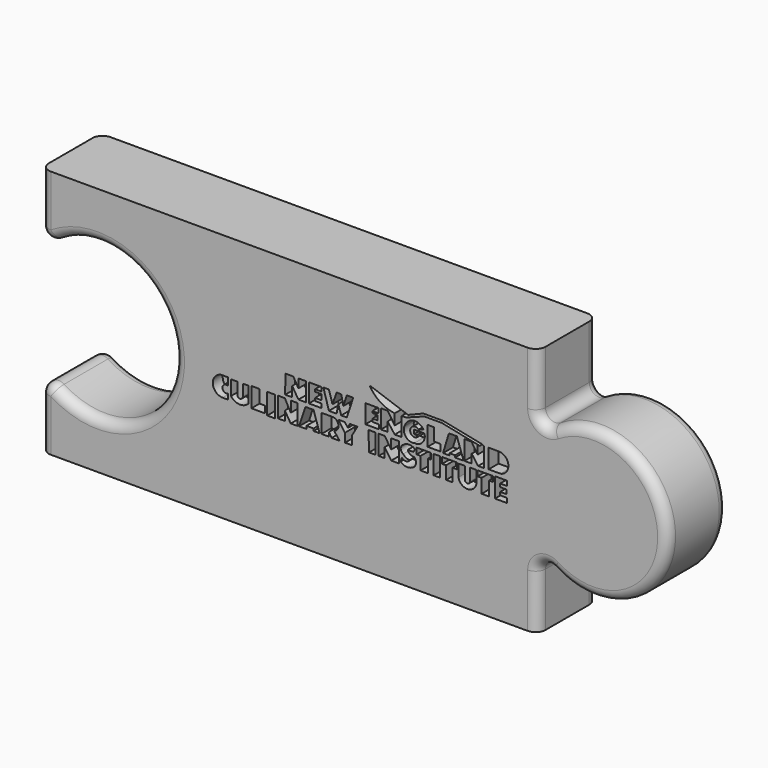
from build123d import *

# Parameters (mm, degrees)
F0_W     = 4.1021890939
F0_H     = 10.701617226
F0_W_2   = 3.2950267196
F0_H_2   = 9.6638526741
F1_DEPTH = 38.1
F2_W     = 160.8449816704
F2_H     = 39.124455303
F3_DEPTH = 31.75
F4_F1_R  = 5.08
F4_F2_R  = 5.08


with BuildPart() as f1:
    # F0 (on Front) → F1 (new body)
    with BuildSketch(Plane.XZ):
        with BuildLine():
            Line((82.5877203729, 87.3429829219), (-171.4122796271, 87.3429829219))
            Line((-171.4122796271, 87.3429829219), (-171.4122796271, 50.2589829219))
            ThreePointArc((-171.4122796271, 50.2589829219), (-103.0818238296, 23.5889829219), (-171.4122796271, -3.0810170781))
            Line((-171.4122796271, -3.0810170781), (-171.4122796271, -40.1650170781))
            Line((-171.4122796271, -40.1650170781), (82.5877203729, -40.1650170781))
            Line((82.5877203729, -40.1650170781), (82.5877203729, -1.8110170781))
            ThreePointArc((82.5877203729, -1.8110170781), (149.0857836871, 23.5889829219), (82.5877203729, 48.9889829219))
            Line((82.5877203729, 48.9889829219), (82.5877203729, 87.3429829219))
        make_face()
        with BuildLine():
            Line((-79.1224884233, 24.1685174963), (-75.8061008891, 24.1685174963))
            Line((-75.8061008891, 24.1685174963), (-75.8061008891, 20.3344915619))
            ThreePointArc((-75.8061008891, 20.3344915619), (-78.5705902931, 18.5480085759), (-75.8061008891, 16.7615255898))
            Line((-75.8061008891, 16.7615255898), (-75.8061008891, 14.1044995373))
            Line((-75.8061008891, 14.1044995373), (-78.4734087428, 14.1044995373))
            ThreePointArc((-78.4734087428, 14.1044995373), (-83.5158724737, 18.8322256207), (-79.1224884233, 24.1685174963))
        make_face(mode=Mode.SUBTRACT)
        with BuildLine():
            Line((-74.1997333607, 16.2316384351), (-74.1997333607, 23.7863697669))
            Line((-74.1997333607, 23.7863697669), (-70.9757404765, 23.7863697669))
            Line((-70.9757404765, 23.7863697669), (-70.9757404765, 18.0120524576))
            ThreePointArc((-70.9757404765, 18.0120524576), (-69.6300867408, 16.5195255788), (-68.1848200402, 17.9158151707))
            Line((-68.1848200402, 17.9158151707), (-68.1848200402, 23.7863697669))
            Line((-68.1848200402, 23.7863697669), (-65.2976604542, 23.7863697669))
            Line((-65.2976604542, 23.7863697669), (-65.2976604542, 15.654207263))
            ThreePointArc((-65.2976604542, 15.654207263), (-69.8819719959, 13.8882631575), (-74.1997333607, 16.2316384351))
        make_face(mode=Mode.SUBTRACT)
        Polygon((-63.7486102423, 14.098005425), (-63.7486102423, 24.1685174963), (-59.7253116211, 24.1685174963), (-59.7253116211, 17.5690884328), (-56.8064423642, 17.5690884328), (-56.8064423642, 14.098005425), align=None, mode=Mode.SUBTRACT)
        with Locations((-53.6509184531, 18.8177088833)):
            Rectangle(F0_W, F0_H, mode=Mode.SUBTRACT)
        Polygon((-46.6518933317, 13.9632076582), (-50.2579296371, 13.9632076582), (-50.2579296371, 24.2781453392), (-46.6518933317, 24.1685174963), (-43.6328882715, 18.6594389936), (-43.6328882715, 24.1685174963), (-40.2784357211, 24.1685174963), (-40.2784357211, 13.7954857758), (-43.6328882715, 13.7954857758), (-46.6518933317, 18.6594389936), align=None, mode=Mode.SUBTRACT)
        Polygon((-31.9960760316, 15.3444652072), (-35.6157990536, 15.3947389311), (-35.6157990536, 13.93679535), (-39.3863441786, 13.93679535), (-36.1185381553, 23.7402115574), (-31.9960760316, 23.7402115574), (-28.8790921113, 14.1881649008), (-31.9960760316, 14.1881649008), align=None, mode=Mode.SUBTRACT)
        with BuildLine():
            Line((-22.6569390288, 14.1316857746), (-24.1320217392, 16.3264675623))
            Line((-24.1320217392, 16.3264675623), (-24.1320217392, 14.2231351322))
            Line((-24.1320217392, 14.2231351322), (-27.91932322, 14.2231351322))
            Line((-27.91932322, 14.2231351322), (-27.91932322, 23.7338562122))
            Line((-27.91932322, 23.7338562122), (-22.2911415985, 23.7338562122))
            ThreePointArc((-22.2911415985, 23.7338562122), (-19.2453874648, 21.0752446961), (-21.4680983117, 17.6982060632))
            Line((-21.4680983117, 17.6982060632), (-18.633171021, 14.1316857746))
            Line((-18.633171021, 14.1316857746), (-22.6569390288, 14.1316857746))
        make_face(mode=Mode.SUBTRACT)
        Polygon((-15.9811424455, 14.1316857746), (-15.9811424455, 18.6126977763), (-19.3647658816, 23.4595090708), (-16.0725927344, 23.4595090708), (-14.3805118641, 21.3320423475), (-13.4205641589, 23.4595090708), (-9.48824644, 23.4595090708), (-12.3231737307, 18.7041480651), (-12.3231737307, 14.2231351322), align=None, mode=Mode.SUBTRACT)
        Polygon((-0.3251792295, 13.8158174789), (-3.5847491017, 13.8158174789), (-3.927862308, 23.8518603703), (-0.3251792295, 23.8518603703), align=None, mode=Mode.SUBTRACT)
        Polygon((4.3926183935, 13.8158174789), (1.3046059394, 13.8158174789), (1.1330493362, 23.8518603703), (4.3926183935, 23.8518603703), (7.7379672657, 18.7909491917), (7.7379672657, 23.8518603703), (11.6837615715, 23.8518603703), (11.6837615715, 13.8158174789), (7.7379672657, 13.8158174789), (4.3926183935, 18.7909491917), align=None, mode=Mode.SUBTRACT)
        with BuildLine():
            ThreePointArc((18.0667647728, 13.9566269329), (15.1280441908, 13.6247220185), (12.455818207, 14.8917846939))
            Line((12.455818207, 14.8917846939), (13.2156335385, 16.9374421796))
            ThreePointArc((13.2156335385, 16.9374421796), (15.2956200346, 15.9580622779), (17.2485019648, 17.1712320855))
            ThreePointArc((17.2485019648, 17.1712320855), (15.3278375039, 17.5219921442), (13.8585548484, 18.8077577016))
            ThreePointArc((13.8585548484, 18.8077577016), (12.5974932093, 20.8534151873), (13.8585548484, 22.899072673))
            ThreePointArc((13.8585548484, 22.899072673), (16.8685940662, 24.0004192145), (19.878633284, 22.899072673))
            Line((19.878633284, 22.899072673), (19.1772654289, 21.3794410786))
            Line((19.1772654289, 21.3794410786), (16.1380022401, 21.3794410786))
            ThreePointArc((16.1380022401, 21.3794410786), (17.4509312815, 19.7687555595), (19.4695023456, 19.2753375134))
            ThreePointArc((19.4695023456, 19.2753375134), (20.2970090792, 16.2127620999), (18.0667647728, 13.9566269329))
        make_face(mode=Mode.SUBTRACT)
        Polygon((22.741639019, 20.7961425743), (20.6964490572, 20.7961425743), (20.6964490572, 23.9033129597), (28.0818557003, 23.9033129597), (28.0818557003, 20.7961425743), (26.4911530176, 20.7961425743), (26.4911530176, 14.2394602856), (22.741639019, 14.2394602856), align=None, mode=Mode.SUBTRACT)
        with Locations((31.0928290346, 19.0713866227)):
            Rectangle(F0_W_2, F0_H_2, mode=Mode.SUBTRACT)
        Polygon((39.1031568506, 14.2394602856), (35.8081282684, 14.2394602856), (35.7312550405, 20.7961425743), (33.7629383066, 20.7961425743), (33.7629383066, 23.8972995988), (41.375587658, 23.8972995988), (41.375587658, 20.7961425743), (39.1031568506, 20.7961425743), align=None, mode=Mode.SUBTRACT)
        with BuildLine():
            Line((42.1253582099, 17.4266091174), (42.1253582099, 23.6942507884))
            Line((42.1253582099, 23.6942507884), (45.3586643198, 23.6942507884))
            Line((45.3586643198, 23.6942507884), (45.3586643198, 17.4266091174))
            ThreePointArc((45.3586643198, 17.4266091174), (46.7496648507, 16.1821081418), (48.0447960654, 17.5260948575))
            Line((48.0447960654, 17.5260948575), (48.0447960654, 23.7937365285))
            Line((48.0447960654, 23.7937365285), (51.2781021753, 23.7937365285))
            Line((51.2781021753, 23.7937365285), (51.2781021753, 17.5260948575))
            ThreePointArc((51.2781021753, 17.5260948575), (46.7430544325, 13.674498706), (42.1253582099, 17.4266091174))
        make_face(mode=Mode.SUBTRACT)
        Polygon((51.9394976655, 21.0886225662), (51.9394976655, 23.8059256783), (59.7690110663, 23.8059256783), (59.7690110663, 21.0886225662), (57.7886020401, 21.0886225662), (57.7886020401, 13.9038926548), (53.9659587303, 13.9038926548), (53.9659587303, 21.0886225662), align=None, mode=Mode.SUBTRACT)
        Polygon((60.7447465518, 13.9480652845), (60.7447465518, 24.0340419671), (63.44380878, 24.0340419671), (66.853153483, 24.0340419671), (66.853153483, 21.6190908661), (63.44380878, 21.6190908661), (63.44380878, 19.9854467621), (66.7111007133, 19.9854467621), (66.7111007133, 17.8546067885), (63.44380878, 17.8546067885), (63.44380878, 16.2919900006), (67.066240088, 16.2919900006), (67.066240088, 13.9480652845), (63.44380878, 13.9480652845), align=None, mode=Mode.SUBTRACT)
        Polygon((-42.9098839304, 25.8483980408), (-46.4937063298, 25.8483980408), (-46.4062684024, 35.39024299), (-42.3295787778, 35.39024299), (-39.7238294026, 30.8894083646), (-39.7238294026, 35.39024299), (-35.9475324294, 35.39024299), (-35.9475324294, 25.8483980408), (-39.7238294026, 25.8483980408), (-42.9098839304, 30.9736058673), align=None, mode=Mode.SUBTRACT)
        Polygon((-34.3518639347, 25.8483980408), (-34.3518639347, 35.39024299), (-27.91932322, 35.39024299), (-27.91932322, 33.288311269), (-31.2072942397, 33.288311269), (-31.2072942397, 32.140087392), (-27.91932322, 32.140087392), (-27.91932322, 29.3885917029), (-31.2072942397, 29.3885917029), (-31.2072942397, 27.9473327658), (-27.91932322, 27.9473327658), (-27.91932322, 25.8483980408), align=None, mode=Mode.SUBTRACT)
        Polygon((-20.2013133457, 25.8483980408), (-24.1320217392, 25.8483980408), (-26.9724550089, 35.4833715221), (-24.1320217392, 35.4833715221), (-22.2976906589, 29.3885917029), (-20.2013133457, 35.39024299), (-17.8428879371, 35.39024299), (-16.7425917825, 30.4357428661), (-14.959094151, 35.8198807201), (-11.6949612638, 35.8198807201), (-14.959094151, 25.8483980408), (-17.8428879371, 25.8483980408), (-19.3337081364, 30.4357428661), align=None, mode=Mode.SUBTRACT)
        Polygon((-5.4699555403, 25.8483980408), (-5.4699555403, 35.39024299), (1.1757765533, 35.39024299), (1.1757765533, 32.9699069819), (-1.9255653387, 32.9699069819), (-1.9255653387, 32.0838094315), (0.6219655843, 32.0838094315), (0.6219655843, 29.6470411679), (-1.8148031449, 29.6470411679), (-1.8148031449, 28.0963704547), (1.5080631347, 28.0963704547), (1.5080631347, 25.8483980408), align=None, mode=Mode.SUBTRACT)
        with BuildLine():
            Line((24.2475764846, 33.265524262), (21.7615682268, 32.337741982))
            ThreePointArc((21.7615682268, 32.337741982), (19.2187327571, 32.9434510536), (17.4847645322, 30.987370815))
            ThreePointArc((17.4847645322, 30.987370815), (18.327813662, 28.655644589), (20.8024000385, 28.5003986767))
            Line((20.8024000385, 28.5003986767), (20.8024000385, 29.5222215912))
            Line((20.8024000385, 29.5222215912), (19.4784858832, 29.5222215912))
            Line((19.4784858832, 29.5222215912), (19.4784858832, 31.5818060747))
            Line((19.4784858832, 31.5818060747), (24.7486075023, 31.5818060747))
            ThreePointArc((24.7486075023, 31.5818060747), (23.7703698462, 27.2257006882), (19.6384498486, 25.5345944872))
            ThreePointArc((19.6384498486, 25.5345944872), (15.2144546519, 26.9788151616), (14.5289026769, 31.5818060747))
            ThreePointArc((14.5289026769, 31.5818060747), (16.4834400671, 34.3767192692), (19.6384498486, 35.6719680688))
            ThreePointArc((19.6384498486, 35.6719680688), (22.2010175105, 34.9629088341), (24.2475764846, 33.265524262))
        make_face(mode=Mode.SUBTRACT)
        with BuildLine():
            ThreePointArc((9.5256541026, 35.6719680688), (2.0934573821, 38.3433933505), (-3.3327658093, 44.0818742475))
            Line((-3.3327658093, 44.0818742475), (16.3243263596, 37.1917598507))
            Line((16.3243263596, 37.1917598507), (24.1828551152, 40.3606482407))
            Line((24.1828551152, 40.3606482407), (34.1483158627, 40.3606482407))
            Line((34.1483158627, 40.3606482407), (54.2648797491, 36.2813287041))
            Line((54.2648797491, 36.2813287041), (55.0723811248, 35.6719680688))
            Line((55.0723811248, 35.6719680688), (55.0723811248, 25.8483980408))
            Line((55.0723811248, 25.8483980408), (52.1580790737, 25.8483980408))
            Line((52.1580790737, 25.8483980408), (48.8858809331, 30.2965418062))
            Line((48.8858809331, 30.2965418062), (48.8858809331, 25.8483980408))
            Line((48.8858809331, 25.8483980408), (45.2046608189, 25.8483980408))
            Line((45.2046608189, 25.8483980408), (45.2046608189, 35.6719680688))
            Line((45.2046608189, 35.6719680688), (48.820163087, 35.6719680688))
            Line((48.820163087, 35.6719680688), (51.9061637679, 30.8592357299))
            Line((51.9061637679, 30.8592357299), (51.9061637679, 35.171344932))
            Line((51.9061637679, 35.171344932), (53.0161512652, 35.171344932))
            Line((53.0161512652, 35.171344932), (33.7054067859, 39.1795598528))
            Line((33.7054067859, 39.1795598528), (24.6995845446, 39.1795598528))
            Line((24.6995845446, 39.1795598528), (15.3009332353, 35.6719680688))
            Line((15.3009332353, 35.6719680688), (13.1191615583, 35.6719680688))
            Line((13.1191615583, 35.6719680688), (13.1191615583, 26.110673379))
            Line((13.1191615583, 26.110673379), (9.5256541026, 26.110673379))
            Line((9.5256541026, 26.110673379), (5.9321474619, 30.8592357299))
            Line((5.9321474619, 30.8592357299), (5.9321474619, 26.110673379))
            Line((5.9321474619, 26.110673379), (2.4669798659, 26.110673379))
            Line((2.4669798659, 26.110673379), (2.4669798659, 35.6719680688))
            Line((2.4669798659, 35.6719680688), (5.9321474619, 35.6719680688))
            Line((5.9321474619, 35.6719680688), (9.5256541026, 30.2175377122))
            Line((9.5256541026, 30.2175377122), (9.5256541026, 35.6719680688))
        make_face(mode=Mode.SUBTRACT)
        Polygon((26.3337166616, 26.062171962), (26.3337166616, 36.0105187258), (29.7282589236, 35.8898193201), (29.7282589236, 29.5049734971), (32.9061699668, 29.5049734971), (32.9061699668, 26.062171962), align=None, mode=Mode.SUBTRACT)
        Polygon((37.5720401862, 25.8092079869), (34.2226167777, 25.8092079869), (37.2411319622, 35.6963053903), (41.2873616079, 35.6963053903), (44.72736545, 25.8092079869), (40.3654304901, 25.8092079869), (40.3654304901, 26.8160794488), (37.5720401862, 26.8160794488), align=None, mode=Mode.SUBTRACT)
        with BuildLine():
            Line((57.5483319917, 26.0820016822), (57.5483319917, 35.8451530895))
            Line((57.5483319917, 35.8451530895), (62.7329153577, 35.8451530895))
            ThreePointArc((62.7329153577, 35.8451530895), (67.6334038948, 31.3574687664), (63.5931631187, 26.0820016822))
            Line((63.5931631187, 26.0820016822), (57.5483319917, 26.0820016822))
        make_face(mode=Mode.SUBTRACT)
    extrude(amount=F1_DEPTH)

    # F2 (on face) → F3 (join)
    with BuildSketch(Plane(origin=(0, 0, 0), x_dir=(-1, 0, 0), z_dir=(0, 1, 0))):
        with Locations((9.6587613225, 28.4752417356)):
            Rectangle(F2_W, F2_H)
    extrude(amount=-F3_DEPTH)

    # F4: fillet of radius 5.08 on 12 edges, made by hand

    # F4_f1
    f4_f1_edges = [f1.edges().sort_by_distance(p)[0] for p in [
        (82.5877203729, -19.05, -1.8110170781),
        (82.5877203729, -19.05, 48.9889829219),
    ]]
    fillet(f4_f1_edges, radius=F4_F1_R)

    # F4_f2
    f4_f2_edges = [f1.edges().sort_by_distance(p)[0] for p in [
        (-171.4122796271, -38.1, 68.8009829219),
        (-171.4122796271, -38.1, -21.6230170781),
        (-103.0818238296, 0, 23.5889829219),
        (-171.4122796271, -19.05, 50.2589829219),
        (-171.4122796271, -19.05, -3.0810170781),
        (-103.0818238296, -38.1, 23.5889829219),
        (-171.4122796271, 0, 68.8009829219),
        (-171.4122796271, 0, -21.6230170781),
        (149.0857836871, 0, 23.5889829219),
        (149.0857836871, -38.1, 23.5889829219),
        (85.2314909048, -38.1, -8.2958477411),
        (85.2314909048, -38.1, 55.473813585),
        (85.2314909048, 0, -8.2958477411),
        (85.2314909048, 0, 55.473813585),
    ]]
    fillet(f4_f2_edges, radius=F4_F2_R)


solid = f1.part
